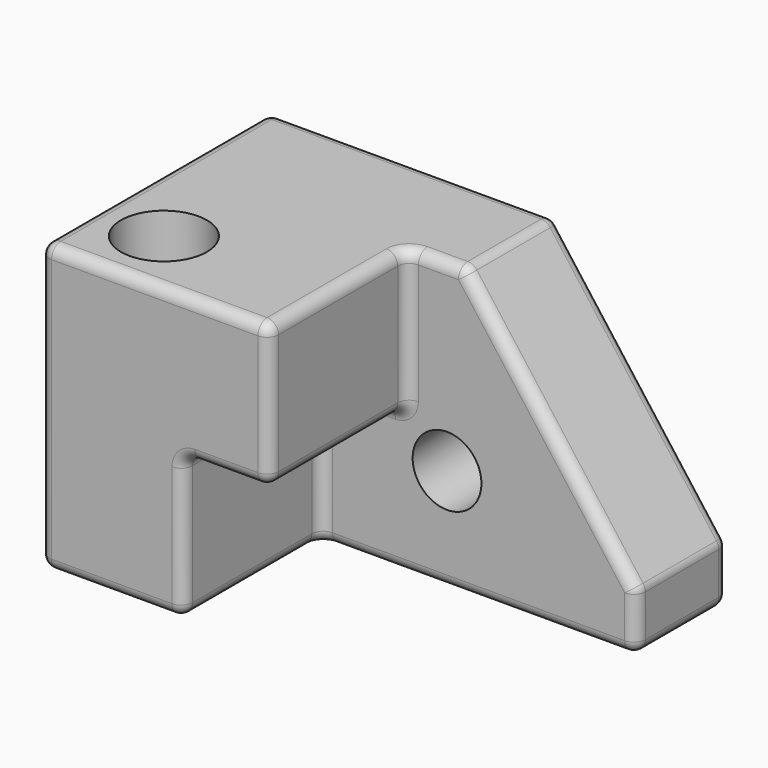
from build123d import *

# Parameters (mm, degrees)
F0_W      = 203.2
F0_H      = 127
F1_DEPTH  = 127
F3_DEPTH  = 76.2
F4_SIZE2  = 101.6
F4_SIZE   = 76.2
F5_R      = 5.08
F7_R      = 15.24
F8_DEPTH  = 50.8
F9_R      = 19.05
F10_DEPTH = 127


# Not quite as in the source:
# - a feature of the source that left no trace in its solid (it failed there, or was rolled back) is left out


with BuildPart() as f1:
    # F0 (on Front) → F1 (new body)
    with BuildSketch(Plane.XZ):
        with Locations((30.3024339037, 3.653427586)):
            Rectangle(F0_W, F0_H)
    extrude(amount=F1_DEPTH)

    # F2 (on face) → F3 (cut)
    with BuildSketch(Plane.XZ.offset(127)):
        Polygon((-7.7975660963, 3.653427586), (-7.7975660963, -59.846572414), (131.9024339037, -59.846572414), (131.9024339037, 67.153427586), (30.3024339037, 67.153427586), (30.3024339037, 3.653427586), align=None)
    extrude(amount=-F3_DEPTH, mode=Mode.SUBTRACT)

    # F4
    f4_edges = [f1.edges().sort_by_distance(p)[0] for p in [
        (131.902434, -25.4, 67.153428),
    ]]
    f4_side = f1.faces().sort_by_distance((8.531005, -52.614286, 67.153428))[0]
    chamfer(f4_edges, length=F4_SIZE, length2=F4_SIZE2, reference=f4_side)

    # F5
    f5_edges = [f1.edges().sort_by_distance(p)[0] for p in [
        (30.302434, -88.9, 67.153428),
        (-20.497566, -127, 67.153428),
        (55.702434, -25.4, 67.153428),
        (131.902434, -25.4, -34.446572),
        (131.902434, -25.4, -59.846572),
        (-39.547566, -127, -59.846572),
        (-7.797566, -88.9, -59.846572),
        (-7.797566, -127, -28.096572),
        (30.302434, -88.9, 3.653428),
        (30.302434, -127, 35.403428),
        (30.302434, -50.8, 35.403428),
        (11.252434, -50.8, 3.653428),
        (-7.797566, -50.8, -28.096572),
        (93.802434, 0, 16.353428),
        (131.902434, 0, -47.146572),
        (-7.797566, 0, 67.153428),
        (30.302434, 0, -59.846572),
        (-71.297566, 0, 3.653428),
        (-71.297566, -63.5, 67.153428),
        (-71.297566, -63.5, -59.846572),
        (131.902434, -50.8, -47.146572),
        (93.802434, -50.8, 16.353428),
        (62.052434, -50.8, -59.846572),
        (43.002434, -50.8, 67.153428),
        (-71.297566, -127, 3.653428),
        (-7.797566, -88.9, 3.653428),
        (11.252434, -127, 3.653428),
    ]]
    fillet(f5_edges, radius=F5_R)

    # F7 (on face) → F8 (cut, through all)
    with BuildSketch(Plane.XZ.offset(50.8)):
        with Locations((48.0824339037, -14.126572414)):
            Circle(F7_R)
    extrude(amount=-F8_DEPTH, mode=Mode.SUBTRACT)

    # F9 (on face) → F10 (cut, through all)
    with BuildSketch(Plane.XY.offset(67.153427586)):
        with Locations((-40.8175660963, -96.52)):
            Circle(F9_R)
    extrude(amount=-F10_DEPTH, mode=Mode.SUBTRACT)


solid = f1.part
